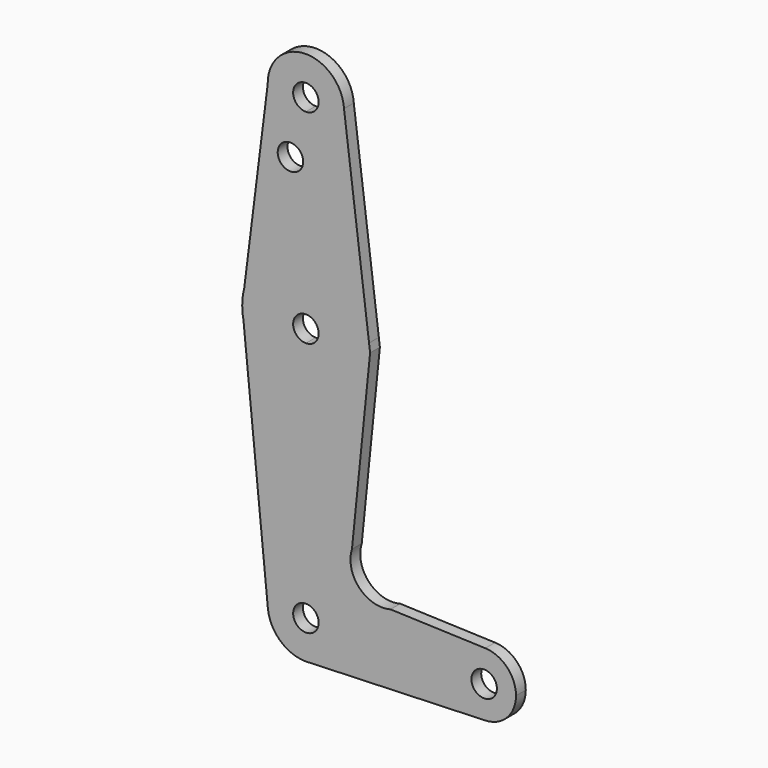
from build123d import *

# Parameters (mm, degrees)
F0_R     = 3.175
F2_DEPTH = 3.048
F4_DEPTH = 3.048


# Not quite as in the source:
# - the program builds the solid bodies; features that only make, move or delete a surface that nothing else refers to are left out


with BuildPart() as f2:
    # F0 (on Front) → F2 (new body)
    with BuildSketch(Plane.XZ):
        with BuildLine():
            ThreePointArc((-53.9726569169, 37.8875110011), (-51.1100820481, 31.2892960094), (-44.45, 28.5737697124))
            ThreePointArc((-44.45, 28.5737697124), (-37.7148079092, 31.3635776216), (-34.925, 38.0987697124))
            ThreePointArc((-34.925, 38.0987697124), (-34.9297776167, 38.4004164794), (-34.9441056739, 38.7017606422))
            ThreePointArc((-34.9441056739, 38.7017606422), (-44.8572110824, 47.6150612241), (-53.9726569169, 37.8875110011))
        make_face()
        with BuildLine():
            ThreePointArc((-41.275, 38.0987697124), (-42.2049359697, 35.8537056822), (-44.45, 34.9237697124))
            ThreePointArc((-44.45, 34.9237697124), (-46.6950640303, 40.3438337427), (-41.275, 38.0987697124))
        make_face(mode=Mode.SUBTRACT)
        with BuildLine():
            ThreePointArc((-34.925, 38.0987697124), (-37.7148079092, 31.3635776216), (-44.45, 28.5737697124))
            Line((-44.45, 28.5737697124), (-44.45, 3.1737697124))
            ThreePointArc((-44.45, 3.1737697124), (-33.9518602832, -0.7930529507), (-28.7002413285, -10.7110728089))
            Line((-28.7002413285, -10.7110728089), (-34.9441056739, 38.7017606422))
            ThreePointArc((-34.9441056739, 38.7017606422), (-34.9297776167, 38.4004164794), (-34.925, 38.0987697124))
        make_face()
        with BuildLine():
            Line((-44.45, 3.1737697124), (-44.45, 28.5737697124))
            ThreePointArc((-44.45, 28.5737697124), (-51.1100820481, 31.2892960094), (-53.9726569169, 37.8875110011))
            Line((-53.9726569169, 37.8875110011), (-59.8162004086, -8.7143129316))
            ThreePointArc((-59.8162004086, -8.7143129316), (-54.1639927932, -0.1451971157), (-44.45, 3.1737697124))
        make_face()
        with Locations((-48.2994141631, 23.748225342)):
            Circle(F0_R, mode=Mode.SUBTRACT)
        with BuildLine():
            ThreePointArc((-28.7002413285, -10.7110728089), (-33.9518602832, -0.7930529507), (-44.45, 3.1737697124))
            Line((-44.45, 3.1737697124), (-44.45, -9.5262302876))
            ThreePointArc((-44.45, -9.5262302876), (-42.2049359697, -10.4561662573), (-41.275, -12.7012302876))
            ThreePointArc((-41.275, -12.7012302876), (-42.2049359697, -14.9462943178), (-44.45, -15.8762302876))
            Line((-44.45, -15.8762302876), (-44.45, -28.5762302876))
            ThreePointArc((-44.45, -28.5762302876), (-33.2246798487, -23.9265504389), (-28.575, -12.7012302876))
            ThreePointArc((-28.575, -12.7012302876), (-28.6063412699, -11.7041831247), (-28.7002413285, -10.7110728089))
        make_face()
        with BuildLine():
            Line((-44.45, -9.5262302876), (-44.45, 3.1737697124))
            ThreePointArc((-44.45, 3.1737697124), (-54.1639927932, -0.1451971157), (-59.8162004086, -8.7143129316))
            Line((-59.8162004086, -8.7143129316), (-60.3248478307, -12.7707382225))
            Line((-60.3248478307, -12.7707382225), (-60.0280973537, -15.7571275106))
            ThreePointArc((-60.0280973537, -15.7571275106), (-54.537201212, -24.959451884), (-44.45, -28.5762302876))
            Line((-44.45, -28.5762302876), (-44.45, -15.8762302876))
            ThreePointArc((-44.45, -15.8762302876), (-47.625, -12.7012302876), (-44.45, -9.5262302876))
        make_face()
        with BuildLine():
            Line((-28.4399795596, -12.7707382225), (-28.7002413285, -10.7110728089))
            ThreePointArc((-28.7002413285, -10.7110728089), (-28.6063412699, -11.7041831247), (-28.575, -12.7012302876))
            ThreePointArc((-28.575, -12.7012302876), (-33.2246798487, -23.9265504389), (-44.45, -28.5762302876))
            Line((-44.45, -28.5762302876), (-44.45, -66.6762302876))
            ThreePointArc((-44.45, -66.6762302876), (-37.7148079092, -69.4660381968), (-34.925, -76.2012302876))
            Line((-34.925, -76.2012302776), (-7.9375, -76.2012302493))
            ThreePointArc((-7.9375, -76.2012302493), (-5.5119104877, -70.48959746), (0.2824052746, -68.2687556265))
            Line((0.2824052746, -68.2687556265), (-23.3412736296, -67.4277253237))
            ThreePointArc((-23.3412736296, -67.4277253237), (-31.1457690986, -65.2277040205), (-32.9607534621, -57.3247884179))
            Line((-32.9607534621, -57.3247884179), (-28.4399795596, -12.7707382225))
        make_face()
        with BuildLine():
            Line((-60.3248478307, -12.7707382225), (-59.8162004086, -8.7143129316))
            ThreePointArc((-59.8162004086, -8.7143129316), (-60.2016481775, -10.7260835353), (-60.3248478307, -12.7707382225))
        make_face()
        with BuildLine():
            Line((-60.0280973537, -15.7571275106), (-60.3248478307, -12.7707382225))
            ThreePointArc((-60.3248478307, -12.7707382225), (-60.2472013483, -14.2709610166), (-60.0280973537, -15.7571275106))
        make_face()
        with BuildLine():
            Line((-44.45, -66.6762302876), (-44.45, -28.5762302876))
            ThreePointArc((-44.45, -28.5762302876), (-54.537201212, -24.959451884), (-60.0280973537, -15.7571275106))
            Line((-60.0280973537, -15.7571275106), (-53.928320809, -77.143068725))
            ThreePointArc((-53.928320809, -77.143068725), (-51.5103341322, -69.8076939467), (-44.45, -66.6762302876))
        make_face()
        with BuildLine():
            Line((-44.45, -73.0262302876), (-44.45, -66.6762302876))
            ThreePointArc((-44.45, -66.6762302876), (-51.5103341322, -69.8076939467), (-53.928320809, -77.143068725))
            ThreePointArc((-53.928320809, -77.143068725), (-50.8924345674, -83.216974143), (-44.5823490099, -85.7253107544))
            Line((-44.5823490099, -85.7253107544), (-43.6430873856, -85.6919898479))
            ThreePointArc((-43.6430873856, -85.6919898479), (-37.4353201195, -82.6448233205), (-34.925, -76.2012302876))
            Line((-34.925, -76.2012302776), (-41.275, -76.2012302842))
            ThreePointArc((-41.275, -76.2012302876), (-46.6950640303, -78.4462943178), (-44.45, -73.0262302876))
        make_face()
        with BuildLine():
            Line((-7.9375, -76.2012302493), (-34.925, -76.2012302776))
            ThreePointArc((-34.925, -76.2012302876), (-37.4353201195, -82.6448233205), (-43.6430873856, -85.6919898479))
            Line((-43.6430873856, -85.6919898479), (0.2814108612, -84.1337401955))
            ThreePointArc((0.2814108612, -84.1337401955), (-5.5122684747, -81.9125175314), (-7.9375, -76.2012302493))
        make_face()
        with BuildLine():
            ThreePointArc((7.9375, -76.201230241), (5.7116327839, -70.6893197563), (0.2824052746, -68.2687556265))
            ThreePointArc((0.2824052746, -68.2687556265), (-5.5119104877, -70.48959746), (-7.9375, -76.2012302493))
            ThreePointArc((-7.9375, -76.2012302493), (-5.5122684747, -81.9125175314), (0.2814108612, -84.1337401955))
            ThreePointArc((0.2814108612, -84.1337401955), (5.7112872875, -81.7134987187), (7.9375, -76.201230241))
        make_face()
        with BuildLine():
            ThreePointArc((3.175, -76.201230241), (1.7e-09, -79.376230241), (-3.175, -76.2012302444))
            ThreePointArc((-3.175, -76.2012302444), (-1.7e-09, -73.026230241), (3.175, -76.201230241))
        make_face(mode=Mode.SUBTRACT)
        with BuildLine():
            Line((-43.6430873856, -85.6919898479), (-44.5823490099, -85.7253107544))
            ThreePointArc((-44.5823490099, -85.7253107544), (-44.1123069666, -85.7202422329), (-43.6430873856, -85.6919898479))
        make_face()
    extrude(amount=F2_DEPTH)

    # F0 (on Front) → F4 (join)
    with BuildSketch(Plane.XZ):
        with BuildLine():
            ThreePointArc((-34.925, -76.2012302876), (-37.7148079092, -69.4660381968), (-44.45, -66.6762302876))
            Line((-44.45, -66.6762302876), (-44.45, -73.0262302876))
            ThreePointArc((-44.45, -73.0262302876), (-42.2049359697, -73.9561662573), (-41.275, -76.2012302876))
            Line((-41.275, -76.2012302842), (-34.925, -76.2012302776))
        make_face()
    extrude(amount=F4_DEPTH)


solid = f2.part
